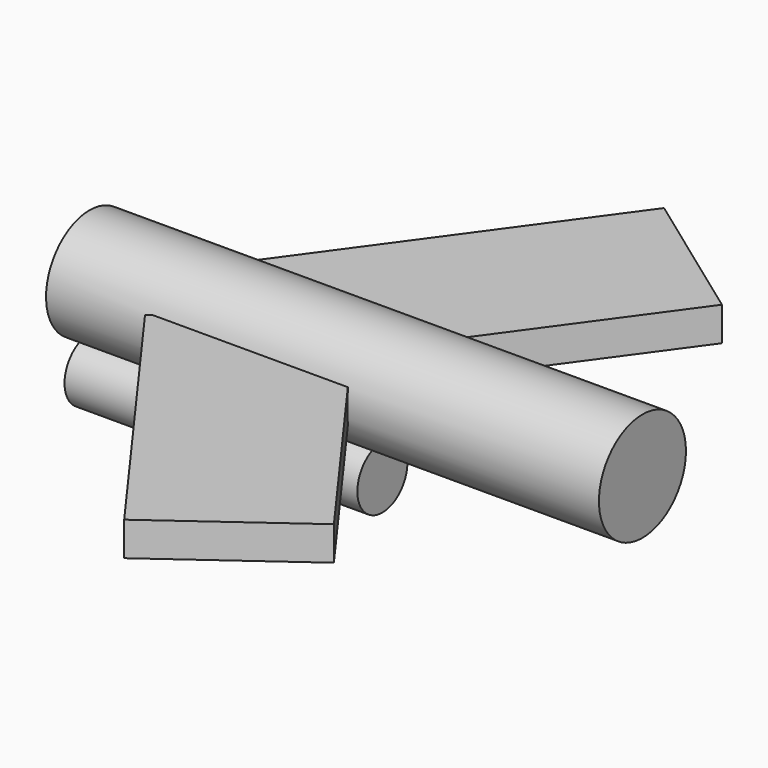
from build123d import *

# Parameters (mm, degrees)
F0_R      = 12.2171028197
F1_DEPTH  = 124.206
F14_R     = 7.0299846098
F15_DEPTH = 65.786
F10_E8_W  = 77.8220303902
F10_E8_H  = 7.62
F16_DEPTH = 36.83
F11_E6_W  = 78.43691694
F11_E6_H  = 7.62
F17_DEPTH = 38.1


# Not quite as in the source:
# - the program builds the solid bodies; features that only make, move or delete a surface that nothing else refers to are left out


with BuildPart() as f1:
    # F0 (on Right) → F1 (new body)
    with BuildSketch(Plane.YZ):
        Circle(F0_R)
    extrude(amount=F1_DEPTH)

    # F14 (on Right) → F15 (join)
    with BuildSketch(Plane.YZ):
        with Locations((0, -19.1768705845)):
            Circle(F14_R)
    extrude(amount=F15_DEPTH)

    # F10_E8 (on explicit) → F16 (join)
    with BuildSketch(Plane(origin=(68.1120529771, -75.4232108593, -3.81), x_dir=(-0.5873196318, 0.8093550828, 0), z_dir=(0.8093550828, 0.5873196318, 0))):
        with Locations((38.9110151951, 3.81)):
            Rectangle(F10_E8_W, F10_E8_H)
    extrude(amount=F16_DEPTH)

    # F11_E6 (on explicit) → F17 (join)
    with BuildSketch(Plane(origin=(68.1120529771, 76.1882886291, -3.81), x_dir=(-0.5862686387, -0.8101167097, 0), z_dir=(-0.8101167097, 0.5862686387, 0))):
        with Locations((39.21845847, 3.81)):
            Rectangle(F11_E6_W, F11_E6_H)
    extrude(amount=-F17_DEPTH)


solid = f1.part
